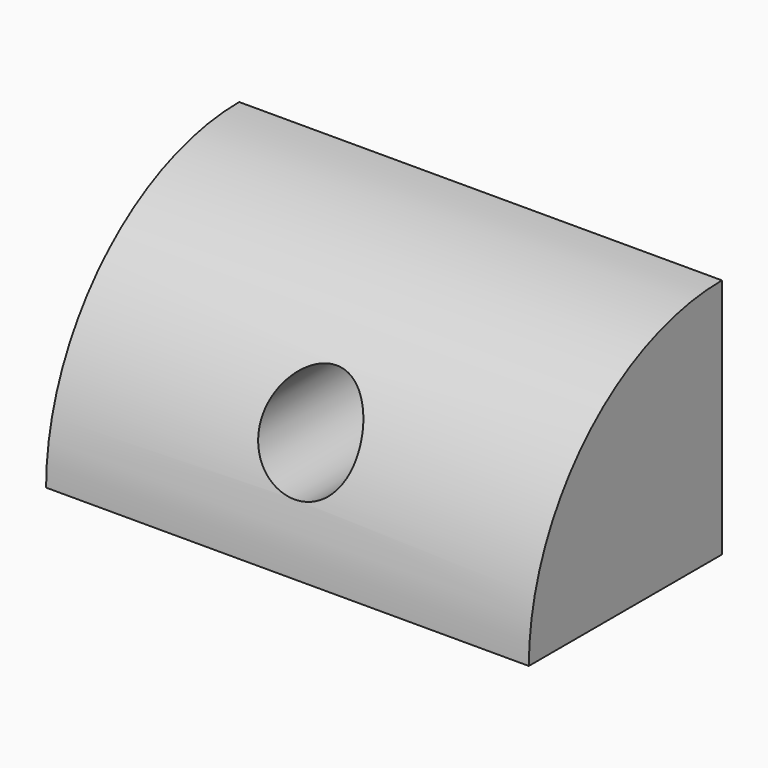
from build123d import *

# Parameters (mm, degrees)
F0_W        = 200
F0_H        = 100
F0_R        = 20
F1_DEPTH    = 100
F2_T1_DEPTH = 700


# Not quite as in the source:
# - a fillet or chamfer that OpenCascade refuses, or shapes differently, is made with other operations: its cross-section is extruded or revolved along the edge and cut away or added


with BuildPart() as f1:
    # F0 (on Front) → F1 (new body)
    with BuildSketch(Plane.XZ):
        Rectangle(F0_W, F0_H)
        with Locations((0, -3.2539968379)):
            Circle(F0_R, mode=Mode.SUBTRACT)
    extrude(amount=F1_DEPTH)

    # F2: fillet of radius 100 on 1 edges, made by hand

    # F2_s2 → F2_t1 (cut)
    with BuildSketch(Plane.YZ.offset(-350)):
        with BuildLine():
            ThreePointArc((0, 50), (-70.7106781187, 20.7106781187), (-100, -50))
            Line((-100, -50), (-100, 50))
            Line((-100, 50), (0, 50))
        make_face()
    extrude(amount=F2_T1_DEPTH, mode=Mode.SUBTRACT)


solid = f1.part
